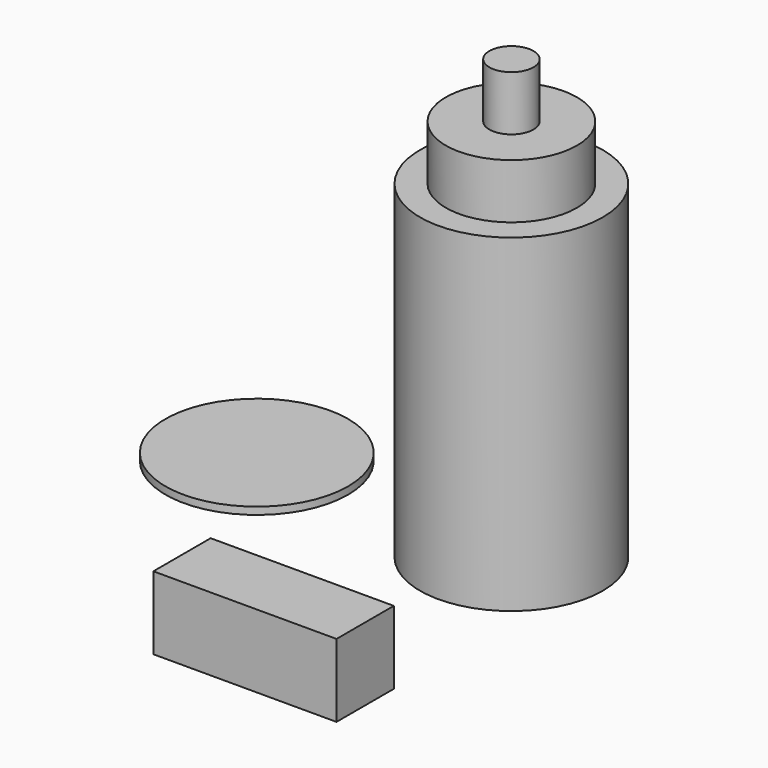
from build123d import *

# Parameters (mm, degrees)
F0_R     = 25
F2_DEPTH = 2
F3_R     = 25
F3_R_2   = 17.9413304425
F4_DEPTH = 90
F3_R_3   = 6.0431477175
F5_DEPTH = 105
F6_DEPTH = 120
F7_W     = 50.1358308829
F7_H     = 19.6019802243
F8_DEPTH = 20


# Not quite as in the source:
# - the program builds the solid bodies; features that only make, move or delete a surface that nothing else refers to are left out


with BuildPart() as f2:
    # F0 (on Top) → F2 (new body)
    with BuildSketch(Plane.XY):
        with Locations((-32.0416949689, 34.2092253268)):
            Circle(F0_R)
    extrude(amount=F2_DEPTH)


with BuildPart() as f4:
    # F3 (on Top) → F4 (new body)
    with BuildSketch(Plane.XY):
        with Locations((38.2615588605, 33.4553010762)):
            Circle(F3_R)
        with Locations((38.2615588605, 33.4553010762)):
            Circle(F3_R_2, mode=Mode.SUBTRACT)
    extrude(amount=F4_DEPTH)

    # F3 (on Top) → F5 (join)
    with BuildSketch(Plane.XY):
        with Locations((38.2615588605, 33.4553010762)):
            Circle(F3_R_2)
        with Locations((38.2615588605, 33.4553010762)):
            Circle(F3_R_3, mode=Mode.SUBTRACT)
    extrude(amount=F5_DEPTH)

    # F3 (on Top) → F6 (join)
    with BuildSketch(Plane.XY):
        with Locations((38.2615588605, 33.4553010762)):
            Circle(F3_R_3)
    extrude(amount=F6_DEPTH)


with BuildPart() as f8:
    # F7 (on Top) → F8 (new body)
    with BuildSketch(Plane.XY):
        with Locations((31.6647354048, -39.6751603112)):
            Rectangle(F7_W, F7_H)
    extrude(amount=F8_DEPTH)


solid = Compound([f2.part, f4.part, f8.part])
